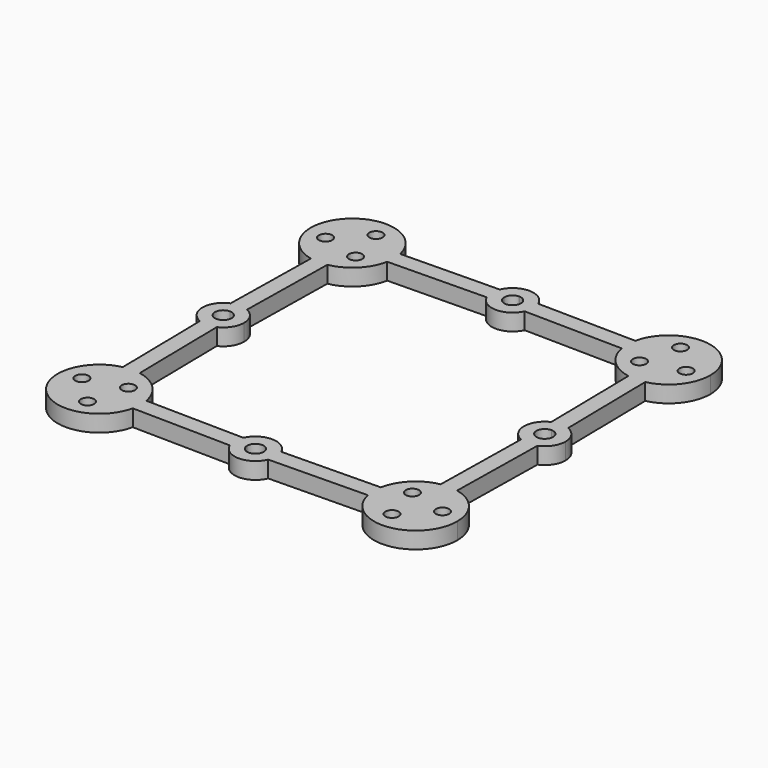
from build123d import *

# Parameters (mm, degrees)
F0_R     = 0.8
F1_DEPTH = 2


with BuildPart() as f1:
    # F0 (on Top) → F1 (new body)
    with BuildSketch(Plane.XY):
        with BuildLine():
            ThreePointArc((17.6211417767, 17.6211417767), (17.7945599777, 17.3616030976), (17.8554563517, 17.0554563517))
            ThreePointArc((17.8554563517, 17.0554563517), (17.3616030976, 16.3163527257), (16.4897709268, 16.4897709268))
            Line((16.4897709268, 16.4897709268), (15.4644660941, 15.4644660941))
            ThreePointArc((15.4644660941, 15.4644660941), (16.6679812638, 14.5771402222), (18.080053157, 14.0853588324))
            Line((18.080053157, 14.0853588324), (18.0159229011, 18.0159229011))
            Line((18.0159229011, 18.0159229011), (17.6211417767, 17.6211417767))
        make_face()
        with BuildLine():
            ThreePointArc((16.4897709268, 16.4897709268), (16.4897709268, 17.6211417767), (17.6211417767, 17.6211417767))
            Line((17.6211417767, 17.6211417767), (18.0159229011, 18.0159229011))
            Line((18.0159229011, 18.0159229011), (14.0853588324, 18.080053157))
            ThreePointArc((14.0853588324, 18.080053157), (14.5771402222, 16.6679812638), (15.4644660941, 15.4644660941))
            Line((15.4644660941, 15.4644660941), (16.4897709268, 16.4897709268))
        make_face()
        with BuildLine():
            Line((14.0853588324, 18.080053157), (18.0159229011, 18.0159229011))
            Line((18.0159229011, 18.0159229011), (19, 19))
            Line((19, 19), (14.0006653796, 19.0815680912))
            ThreePointArc((14.0006653796, 19.0815680912), (14.017782921, 18.5786771094), (14.0853588324, 18.080053157))
        make_face()
        with BuildLine():
            Line((19, 19), (18.0159229011, 18.0159229011))
            Line((18.0159229011, 18.0159229011), (18.080053157, 14.0853588324))
            ThreePointArc((18.080053157, 14.0853588324), (18.5786771094, 14.017782921), (19.0815680912, 14.0006653796))
            Line((19.0815680912, 14.0006653796), (19, 19))
        make_face()
        with BuildLine():
            Line((14.0006653796, 19.0815680912), (19, 19))
            Line((19, 19), (19.0815680912, 14.0006653796))
            ThreePointArc((19.0815680912, 14.0006653796), (19.5836329763, 14.0341795694), (20.0797870051, 14.1179860689))
            Line((20.0797870051, 14.1179860689), (19.9840770989, 19.9840770989))
            Line((19.9840770989, 19.9840770989), (14.1179860689, 20.0797870051))
            ThreePointArc((14.1179860689, 20.0797870051), (14.0341795694, 19.5836329763), (14.0006653796, 19.0815680912))
        make_face()
        with BuildLine():
            Line((2.274669314, 18.2727538807), (14.0853588324, 18.080053157))
            ThreePointArc((14.0853588324, 18.080053157), (14.017782921, 18.5786771094), (14.0006653796, 19.0815680912))
            Line((14.0006653796, 19.0815680912), (2.4996673102, 19.2692159544))
            ThreePointArc((2.4996673102, 19.2692159544), (2.4386075363, 18.7593701028), (2.274669314, 18.2727538807))
        make_face()
        with BuildLine():
            ThreePointArc((19.0815680912, 14.0006653796), (18.5786771094, 14.017782921), (18.080053157, 14.0853588324))
            Line((18.080053157, 14.0853588324), (18.2727538807, 2.274669314))
            ThreePointArc((18.2727538807, 2.274669314), (18.7593701028, 2.4386075363), (19.2692159544, 2.4996673102))
            Line((19.2692159544, 2.4996673102), (19.0815680912, 14.0006653796))
        make_face()
        with BuildLine():
            ThreePointArc((20.0797870051, 14.1179860689), (19.5836329763, 14.0341795694), (19.0815680912, 14.0006653796))
            Line((19.0815680912, 14.0006653796), (19.2692159544, 2.4996673102))
            ThreePointArc((19.2692159544, 2.4996673102), (19.7807823778, 2.455272684), (20.2724877289, 2.3072965505))
            Line((20.2724877289, 2.3072965505), (20.0797870051, 14.1179860689))
        make_face()
        with BuildLine():
            Line((2.4996673102, 19.2692159544), (14.0006653796, 19.0815680912))
            ThreePointArc((14.0006653796, 19.0815680912), (14.0341795694, 19.5836329763), (14.1179860689, 20.0797870051))
            Line((14.1179860689, 20.0797870051), (2.3072965505, 20.2724877289))
            ThreePointArc((2.3072965505, 20.2724877289), (2.4513507885, 19.800794572), (2.5, 19.31))
            ThreePointArc((2.5, 19.31), (2.4999168262, 19.2896072988), (2.4996673102, 19.2692159544))
        make_face()
        with BuildLine():
            Line((0, 18.3098669064), (2.274669314, 18.2727538807))
            ThreePointArc((2.274669314, 18.2727538807), (2.4386075363, 18.7593701028), (2.4996673102, 19.2692159544))
            Line((2.4996673102, 19.2692159544), (0.9998669241, 19.2936863818))
            ThreePointArc((0.9998669241, 19.2936863818), (0, 18.31), (-0.9998669241, 19.2936863818))
            Line((-0.9998669241, 19.2936863818), (-2.4996673102, 19.2692159544))
            ThreePointArc((-2.4996673102, 19.2692159544), (-2.4386075363, 18.7593701028), (-2.274669314, 18.2727538807))
            Line((-2.274669314, 18.2727538807), (0, 18.3098669064))
        make_face()
        with BuildLine():
            ThreePointArc((-2.274669314, 18.2727538807), (0, 16.81), (2.274669314, 18.2727538807))
            Line((2.274669314, 18.2727538807), (0, 18.3098669064))
            Line((0, 18.3098669064), (-2.274669314, 18.2727538807))
        make_face()
        with BuildLine():
            Line((18.3098669064, 0), (18.2727538807, 2.274669314))
            ThreePointArc((18.2727538807, 2.274669314), (16.81, 0), (18.2727538807, -2.274669314))
            Line((18.2727538807, -2.274669314), (18.3098669064, 0))
        make_face()
        with BuildLine():
            ThreePointArc((19.2692159544, 2.4996673102), (18.7593701028, 2.4386075363), (18.2727538807, 2.274669314))
            Line((18.2727538807, 2.274669314), (18.3098669064, 0))
            Line((18.3098669064, 0), (18.2727538807, -2.274669314))
            ThreePointArc((18.2727538807, -2.274669314), (18.7593701028, -2.4386075363), (19.2692159544, -2.4996673102))
            Line((19.2692159544, -2.4996673102), (19.2936863818, -0.9998669241))
            ThreePointArc((19.2936863818, -0.9998669241), (18.31, 0), (19.2936863818, 0.9998669241))
            Line((19.2936863818, 0.9998669241), (19.2692159544, 2.4996673102))
        make_face()
        with BuildLine():
            Line((19.9840770989, 19.9840770989), (20.0797870051, 14.1179860689))
            ThreePointArc((20.0797870051, 14.1179860689), (22.8986494473, 15.8694197843), (24, 19))
            ThreePointArc((24, 19), (19.5431069621, 23.9704159612), (14.1179860689, 20.0797870051))
            Line((14.1179860689, 20.0797870051), (19.9840770989, 19.9840770989))
        make_face()
        with Locations((21.6562960223, 18.288247626)):
            Circle(F0_R, mode=Mode.SUBTRACT)
        with Locations((18.288247626, 21.6562960223)):
            Circle(F0_R, mode=Mode.SUBTRACT)
        with BuildLine():
            ThreePointArc((20.2724877289, 2.3072965505), (19.7807823778, 2.455272684), (19.2692159544, 2.4996673102))
            Line((19.2692159544, 2.4996673102), (19.2936863818, 0.9998669241))
            ThreePointArc((19.2936863818, 0.9998669241), (20.0054772146, 0.7185481501), (20.3098669242, 0.0163136116))
            Line((20.3098669242, 0.0163136116), (20.2724877289, 2.3072965505))
        make_face()
        with BuildLine():
            Line((0.9998669241, 19.2936863818), (2.4996673102, 19.2692159544))
            ThreePointArc((2.4996673102, 19.2692159544), (2.4999168262, 19.2896072988), (2.5, 19.31))
            ThreePointArc((2.5, 19.31), (2.4513507885, 19.800794572), (2.3072965505, 20.2724877289))
            Line((2.3072965505, 20.2724877289), (0.0163136221, 20.309866924))
            ThreePointArc((0.0163136221, 20.309866924), (0.7128511844, 20.0113153278), (1, 19.31))
            ThreePointArc((1, 19.31), (0.9999667305, 19.3018429195), (0.9998669241, 19.2936863818))
        make_face()
        with BuildLine():
            Line((-14.0853588324, 18.080053157), (-2.274669314, 18.2727538807))
            ThreePointArc((-2.274669314, 18.2727538807), (-2.4386075363, 18.7593701028), (-2.4996673102, 19.2692159544))
            Line((-2.4996673102, 19.2692159544), (-14.0006653796, 19.0815680912))
            ThreePointArc((-14.0006653796, 19.0815680912), (-14.0001663477, 19.0407854025), (-14, 19))
            ThreePointArc((-14, 19), (-14.0213854418, 18.5380507809), (-14.0853588324, 18.080053157))
        make_face()
        with BuildLine():
            ThreePointArc((19.2692159544, -2.4996673102), (18.7593701028, -2.4386075363), (18.2727538807, -2.274669314))
            Line((18.2727538807, -2.274669314), (18.080053157, -14.0853588324))
            ThreePointArc((18.080053157, -14.0853588324), (18.5786771094, -14.017782921), (19.0815680912, -14.0006653796))
            Line((19.0815680912, -14.0006653796), (19.2692159544, -2.4996673102))
        make_face()
        with BuildLine():
            ThreePointArc((21.81, 0), (21.3904109356, 1.3863225955), (20.2724877289, 2.3072965505))
            Line((20.2724877289, 2.3072965505), (20.3098669242, 0.0163136116))
            Line((20.3098669242, 0.0163136116), (20.3101330936, 0))
            Line((20.3101330936, 0), (20.3098669233, -0.0163136677))
            Line((20.3098669233, -0.0163136677), (20.2724877289, -2.3072965505))
            ThreePointArc((20.2724877289, -2.3072965505), (21.3904109356, -1.3863225955), (21.81, 0))
        make_face()
        with BuildLine():
            Line((0.0163136221, 20.309866924), (2.3072965505, 20.2724877289))
            ThreePointArc((2.3072965505, 20.2724877289), (0, 21.81), (-2.3072965505, 20.2724877289))
            Line((-2.3072965505, 20.2724877289), (-0.0163136221, 20.309866924))
            Line((-0.0163136221, 20.309866924), (0, 20.3101330936))
            Line((0, 20.3101330936), (0.0163136221, 20.309866924))
        make_face()
        with BuildLine():
            Line((-14.0006653796, 19.0815680912), (-2.4996673102, 19.2692159544))
            ThreePointArc((-2.4996673102, 19.2692159544), (-2.455272684, 19.7807823778), (-2.3072965505, 20.2724877289))
            Line((-2.3072965505, 20.2724877289), (-14.1179860689, 20.0797870051))
            ThreePointArc((-14.1179860689, 20.0797870051), (-14.0341795694, 19.5836329763), (-14.0006653796, 19.0815680912))
        make_face()
        with BuildLine():
            ThreePointArc((-2.3072965505, 20.2724877289), (-2.455272684, 19.7807823778), (-2.4996673102, 19.2692159544))
            Line((-2.4996673102, 19.2692159544), (-0.9998669241, 19.2936863818))
            ThreePointArc((-0.9998669241, 19.2936863818), (-0.7185481537, 20.0054772108), (-0.0163136221, 20.309866924))
            Line((-0.0163136221, 20.309866924), (-2.3072965505, 20.2724877289))
        make_face()
        with BuildLine():
            Line((-18.0159229011, 18.0159229011), (-14.0853588324, 18.080053157))
            ThreePointArc((-14.0853588324, 18.080053157), (-14.0213854418, 18.5380507809), (-14, 19))
            ThreePointArc((-14, 19), (-14.0001663477, 19.0407854025), (-14.0006653796, 19.0815680912))
            Line((-14.0006653796, 19.0815680912), (-19, 19))
            Line((-19, 19), (-19.0815680912, 14.0006653796))
            ThreePointArc((-19.0815680912, 14.0006653796), (-18.5786771094, 14.017782921), (-18.080053157, 14.0853588324))
            Line((-18.080053157, 14.0853588324), (-18.0159229011, 18.0159229011))
        make_face()
        with BuildLine():
            ThreePointArc((-18.080053157, 14.0853588324), (-15.4644660941, 15.4644660941), (-14.0853588324, 18.080053157))
            Line((-14.0853588324, 18.080053157), (-18.0159229011, 18.0159229011))
            Line((-18.0159229011, 18.0159229011), (-18.080053157, 14.0853588324))
        make_face()
        with Locations((-17.0554563517, 17.0554563517)):
            Circle(F0_R, mode=Mode.SUBTRACT)
        with BuildLine():
            Line((19.2936863818, -0.9998669241), (19.2692159544, -2.4996673102))
            ThreePointArc((19.2692159544, -2.4996673102), (19.7807823778, -2.455272684), (20.2724877289, -2.3072965505))
            Line((20.2724877289, -2.3072965505), (20.3098669233, -0.0163136677))
            ThreePointArc((20.3098669233, -0.0163136677), (20.0054771945, -0.7185481696), (19.2936863818, -0.9998669241))
        make_face()
        with BuildLine():
            ThreePointArc((20.2724877289, -2.3072965505), (19.7807823778, -2.455272684), (19.2692159544, -2.4996673102))
            Line((19.2692159544, -2.4996673102), (19.0815680912, -14.0006653796))
            ThreePointArc((19.0815680912, -14.0006653796), (19.5836329763, -14.0341795694), (20.0797870051, -14.1179860689))
            Line((20.0797870051, -14.1179860689), (20.2724877289, -2.3072965505))
        make_face()
        with BuildLine():
            Line((18.0159229011, -18.0159229011), (18.080053157, -14.0853588324))
            ThreePointArc((18.080053157, -14.0853588324), (15.4644660941, -15.4644660941), (14.0853588324, -18.080053157))
            Line((14.0853588324, -18.080053157), (18.0159229011, -18.0159229011))
        make_face()
        with Locations((17.0554563517, -17.0554563517)):
            Circle(F0_R, mode=Mode.SUBTRACT)
        with BuildLine():
            ThreePointArc((19.0815680912, -14.0006653796), (18.5786771094, -14.017782921), (18.080053157, -14.0853588324))
            Line((18.080053157, -14.0853588324), (18.0159229011, -18.0159229011))
            Line((18.0159229011, -18.0159229011), (14.0853588324, -18.080053157))
            ThreePointArc((14.0853588324, -18.080053157), (14.017782921, -18.5786771094), (14.0006653796, -19.0815680912))
            Line((14.0006653796, -19.0815680912), (19, -19))
            Line((19, -19), (19.0815680912, -14.0006653796))
        make_face()
        with BuildLine():
            Line((20.3101330936, 0), (20.3098669242, 0.0163136116))
            ThreePointArc((20.3098669242, 0.0163136116), (20.3099667305, 0.0081570772), (20.31, 0))
            ThreePointArc((20.31, 0), (20.3099667303, -0.0081571052), (20.3098669233, -0.0163136677))
            Line((20.3098669233, -0.0163136677), (20.3101330936, 0))
        make_face()
        with BuildLine():
            ThreePointArc((-0.0163136221, 20.309866924), (0, 20.31), (0.0163136221, 20.309866924))
            Line((0.0163136221, 20.309866924), (0, 20.3101330936))
            Line((0, 20.3101330936), (-0.0163136221, 20.309866924))
        make_face()
        with BuildLine():
            Line((-19, 19), (-14.0006653796, 19.0815680912))
            ThreePointArc((-14.0006653796, 19.0815680912), (-14.0341795694, 19.5836329763), (-14.1179860689, 20.0797870051))
            ThreePointArc((-14.1179860689, 20.0797870051), (-22.5355339059, 22.5355339059), (-20.0797870051, 14.1179860689))
            ThreePointArc((-20.0797870051, 14.1179860689), (-19.5836329763, 14.0341795694), (-19.0815680912, 14.0006653796))
            Line((-19.0815680912, 14.0006653796), (-19, 19))
        make_face()
        with Locations((-21.6562960223, 18.288247626)):
            Circle(F0_R, mode=Mode.SUBTRACT)
        with Locations((-18.288247626, 21.6562960223)):
            Circle(F0_R, mode=Mode.SUBTRACT)
        with BuildLine():
            Line((-18.2727538807, 2.274669314), (-18.080053157, 14.0853588324))
            ThreePointArc((-18.080053157, 14.0853588324), (-18.5786771094, 14.017782921), (-19.0815680912, 14.0006653796))
            Line((-19.0815680912, 14.0006653796), (-19.2692159544, 2.4996673102))
            ThreePointArc((-19.2692159544, 2.4996673102), (-18.7593701028, 2.4386075363), (-18.2727538807, 2.274669314))
        make_face()
        with BuildLine():
            ThreePointArc((20.0797870051, -14.1179860689), (19.5836329763, -14.0341795694), (19.0815680912, -14.0006653796))
            Line((19.0815680912, -14.0006653796), (19, -19))
            Line((19, -19), (14.0006653796, -19.0815680912))
            ThreePointArc((14.0006653796, -19.0815680912), (14.0341795694, -19.5836329763), (14.1179860689, -20.0797870051))
            Line((14.1179860689, -20.0797870051), (19.9840770989, -19.9840770989))
            Line((19.9840770989, -19.9840770989), (20.0797870051, -14.1179860689))
        make_face()
        with BuildLine():
            ThreePointArc((14.0006653796, -19.0815680912), (14.017782921, -18.5786771094), (14.0853588324, -18.080053157))
            Line((14.0853588324, -18.080053157), (2.274669314, -18.2727538807))
            ThreePointArc((2.274669314, -18.2727538807), (2.4386075363, -18.7593701028), (2.4996673102, -19.2692159544))
            Line((2.4996673102, -19.2692159544), (14.0006653796, -19.0815680912))
        make_face()
        with BuildLine():
            Line((-19.2692159544, 2.4996673102), (-19.0815680912, 14.0006653796))
            ThreePointArc((-19.0815680912, 14.0006653796), (-19.5836329763, 14.0341795694), (-20.0797870051, 14.1179860689))
            Line((-20.0797870051, 14.1179860689), (-20.2724877289, 2.3072965505))
            ThreePointArc((-20.2724877289, 2.3072965505), (-19.7807823778, 2.455272684), (-19.2692159544, 2.4996673102))
        make_face()
        with BuildLine():
            ThreePointArc((-16.81, 0), (-17.2072499794, 1.3521990796), (-18.2727538807, 2.274669314))
            ThreePointArc((-18.2727538807, 2.274669314), (-18.7593701028, 2.4386075363), (-19.2692159544, 2.4996673102))
            Line((-19.2692159544, 2.4996673102), (-19.2936863818, 0.9998669241))
            ThreePointArc((-19.2936863818, 0.9998669241), (-18.597148817, 0.7013153291), (-18.31, 0))
            ThreePointArc((-18.31, 0), (-18.597148817, -0.7013153291), (-19.2936863818, -0.9998669241))
            Line((-19.2936863818, -0.9998669241), (-19.2692159544, -2.4996673102))
            ThreePointArc((-19.2692159544, -2.4996673102), (-18.7593701028, -2.4386075363), (-18.2727538807, -2.274669314))
            ThreePointArc((-18.2727538807, -2.274669314), (-17.2072499794, -1.3521990796), (-16.81, 0))
        make_face()
        with BuildLine():
            ThreePointArc((24, -19), (22.8986494473, -15.8694197843), (20.0797870051, -14.1179860689))
            Line((20.0797870051, -14.1179860689), (19.9840770989, -19.9840770989))
            Line((19.9840770989, -19.9840770989), (14.1179860689, -20.0797870051))
            ThreePointArc((14.1179860689, -20.0797870051), (19.5431069621, -23.9704159612), (24, -19))
        make_face()
        with Locations((18.288247626, -21.6562960223)):
            Circle(F0_R, mode=Mode.SUBTRACT)
        with Locations((21.6562960223, -18.288247626)):
            Circle(F0_R, mode=Mode.SUBTRACT)
        with BuildLine():
            ThreePointArc((14.1179860689, -20.0797870051), (14.0341795694, -19.5836329763), (14.0006653796, -19.0815680912))
            Line((14.0006653796, -19.0815680912), (2.4996673102, -19.2692159544))
            ThreePointArc((2.4996673102, -19.2692159544), (2.4999168262, -19.2896072988), (2.5, -19.31))
            ThreePointArc((2.5, -19.31), (2.4513507885, -19.800794572), (2.3072965505, -20.2724877289))
            Line((2.3072965505, -20.2724877289), (14.1179860689, -20.0797870051))
        make_face()
        with BuildLine():
            Line((0, -18.3098669064), (2.274669314, -18.2727538807))
            ThreePointArc((2.274669314, -18.2727538807), (0, -16.81), (-2.274669314, -18.2727538807))
            Line((-2.274669314, -18.2727538807), (0, -18.3098669064))
        make_face()
        with BuildLine():
            ThreePointArc((2.4996673102, -19.2692159544), (2.4386075363, -18.7593701028), (2.274669314, -18.2727538807))
            Line((2.274669314, -18.2727538807), (0, -18.3098669064))
            Line((0, -18.3098669064), (-2.274669314, -18.2727538807))
            ThreePointArc((-2.274669314, -18.2727538807), (-2.4386075363, -18.7593701028), (-2.4996673102, -19.2692159544))
            Line((-2.4996673102, -19.2692159544), (-0.9998669241, -19.2936863818))
            ThreePointArc((-0.9998669241, -19.2936863818), (0, -18.31), (0.9998669241, -19.2936863818))
            Line((0.9998669241, -19.2936863818), (2.4996673102, -19.2692159544))
        make_face()
        with BuildLine():
            Line((-19.2936863818, 0.9998669241), (-19.2692159544, 2.4996673102))
            ThreePointArc((-19.2692159544, 2.4996673102), (-19.7807823778, 2.455272684), (-20.2724877289, 2.3072965505))
            ThreePointArc((-20.2724877289, 2.3072965505), (-21.81, 0), (-20.2724877289, -2.3072965505))
            ThreePointArc((-20.2724877289, -2.3072965505), (-19.7807823778, -2.455272684), (-19.2692159544, -2.4996673102))
            Line((-19.2692159544, -2.4996673102), (-19.2936863818, -0.9998669241))
            ThreePointArc((-19.2936863818, -0.9998669241), (-20.31, 0), (-19.2936863818, 0.9998669241))
        make_face()
        with BuildLine():
            ThreePointArc((2.5, -19.31), (2.4999168262, -19.2896072988), (2.4996673102, -19.2692159544))
            Line((2.4996673102, -19.2692159544), (0.9998669241, -19.2936863818))
            ThreePointArc((0.9998669241, -19.2936863818), (0.9999667305, -19.3018429195), (1, -19.31))
            ThreePointArc((1, -19.31), (0.7128511844, -20.0113153278), (0.0163136221, -20.309866924))
            Line((0.0163136221, -20.309866924), (2.3072965505, -20.2724877289))
            ThreePointArc((2.3072965505, -20.2724877289), (2.4513507885, -19.800794572), (2.5, -19.31))
        make_face()
        with BuildLine():
            ThreePointArc((-2.4996673102, -19.2692159544), (-2.4386075363, -18.7593701028), (-2.274669314, -18.2727538807))
            Line((-2.274669314, -18.2727538807), (-14.0853588324, -18.080053157))
            ThreePointArc((-14.0853588324, -18.080053157), (-14.0213854418, -18.5380507809), (-14, -19))
            ThreePointArc((-14, -19), (-14.0001663477, -19.0407854025), (-14.0006653796, -19.0815680912))
            Line((-14.0006653796, -19.0815680912), (-2.4996673102, -19.2692159544))
        make_face()
        with BuildLine():
            Line((-18.080053157, -14.0853588324), (-18.2727538807, -2.274669314))
            ThreePointArc((-18.2727538807, -2.274669314), (-18.7593701028, -2.4386075363), (-19.2692159544, -2.4996673102))
            Line((-19.2692159544, -2.4996673102), (-19.0815680912, -14.0006653796))
            ThreePointArc((-19.0815680912, -14.0006653796), (-18.5786771094, -14.017782921), (-18.080053157, -14.0853588324))
        make_face()
        with BuildLine():
            ThreePointArc((-2.3072965505, -20.2724877289), (0, -21.81), (2.3072965505, -20.2724877289))
            Line((2.3072965505, -20.2724877289), (0.0163136221, -20.309866924))
            Line((0.0163136221, -20.309866924), (0, -20.3101330936))
            Line((0, -20.3101330936), (-0.0163136391, -20.3098669237))
            Line((-0.0163136391, -20.3098669237), (-2.3072965505, -20.2724877289))
        make_face()
        with BuildLine():
            Line((-0.9998669241, -19.2936863818), (-2.4996673102, -19.2692159544))
            ThreePointArc((-2.4996673102, -19.2692159544), (-2.455272684, -19.7807823778), (-2.3072965505, -20.2724877289))
            Line((-2.3072965505, -20.2724877289), (-0.0163136391, -20.3098669237))
            ThreePointArc((-0.0163136391, -20.3098669237), (-0.7185481596, -20.0054772047), (-0.9998669241, -19.2936863818))
        make_face()
        with BuildLine():
            ThreePointArc((-2.3072965505, -20.2724877289), (-2.455272684, -19.7807823778), (-2.4996673102, -19.2692159544))
            Line((-2.4996673102, -19.2692159544), (-14.0006653796, -19.0815680912))
            ThreePointArc((-14.0006653796, -19.0815680912), (-14.0341795694, -19.5836329763), (-14.1179860689, -20.0797870051))
            Line((-14.1179860689, -20.0797870051), (-2.3072965505, -20.2724877289))
        make_face()
        with BuildLine():
            Line((-18.0159229011, -18.0159229011), (-14.0853588324, -18.080053157))
            ThreePointArc((-14.0853588324, -18.080053157), (-15.4644660941, -15.4644660941), (-18.080053157, -14.0853588324))
            Line((-18.080053157, -14.0853588324), (-18.0159229011, -18.0159229011))
        make_face()
        with Locations((-17.0554563517, -17.0554563517)):
            Circle(F0_R, mode=Mode.SUBTRACT)
        with BuildLine():
            ThreePointArc((-14, -19), (-14.0213854418, -18.5380507809), (-14.0853588324, -18.080053157))
            Line((-14.0853588324, -18.080053157), (-18.0159229011, -18.0159229011))
            Line((-18.0159229011, -18.0159229011), (-18.080053157, -14.0853588324))
            ThreePointArc((-18.080053157, -14.0853588324), (-18.5786771094, -14.017782921), (-19.0815680912, -14.0006653796))
            Line((-19.0815680912, -14.0006653796), (-19, -19))
            Line((-19, -19), (-14.0006653796, -19.0815680912))
            ThreePointArc((-14.0006653796, -19.0815680912), (-14.0001663477, -19.0407854025), (-14, -19))
        make_face()
        with BuildLine():
            ThreePointArc((-19.2692159544, -2.4996673102), (-19.7807823778, -2.455272684), (-20.2724877289, -2.3072965505))
            Line((-20.2724877289, -2.3072965505), (-20.0797870051, -14.1179860689))
            ThreePointArc((-20.0797870051, -14.1179860689), (-19.5836329763, -14.0341795694), (-19.0815680912, -14.0006653796))
            Line((-19.0815680912, -14.0006653796), (-19.2692159544, -2.4996673102))
        make_face()
        with BuildLine():
            Line((0, -20.3101330936), (0.0163136221, -20.309866924))
            ThreePointArc((0.0163136221, -20.309866924), (-8.5e-09, -20.31), (-0.0163136391, -20.3098669237))
            Line((-0.0163136391, -20.3098669237), (0, -20.3101330936))
        make_face()
        with BuildLine():
            ThreePointArc((-14.1179860689, -20.0797870051), (-14.0341795694, -19.5836329763), (-14.0006653796, -19.0815680912))
            Line((-14.0006653796, -19.0815680912), (-19, -19))
            Line((-19, -19), (-19.0815680912, -14.0006653796))
            ThreePointArc((-19.0815680912, -14.0006653796), (-19.5836329763, -14.0341795694), (-20.0797870051, -14.1179860689))
            Line((-20.0797870051, -14.1179860689), (-19.9840770989, -19.9840770989))
            Line((-19.9840770989, -19.9840770989), (-14.1179860689, -20.0797870051))
        make_face()
        with BuildLine():
            Line((-19.9840770989, -19.9840770989), (-20.0797870051, -14.1179860689))
            ThreePointArc((-20.0797870051, -14.1179860689), (-22.5355339059, -22.5355339059), (-14.1179860689, -20.0797870051))
            Line((-14.1179860689, -20.0797870051), (-19.9840770989, -19.9840770989))
        make_face()
        with Locations((-18.288247626, -21.6562960223)):
            Circle(F0_R, mode=Mode.SUBTRACT)
        with Locations((-21.6562960223, -18.288247626)):
            Circle(F0_R, mode=Mode.SUBTRACT)
    extrude(amount=F1_DEPTH)


solid = f1.part
